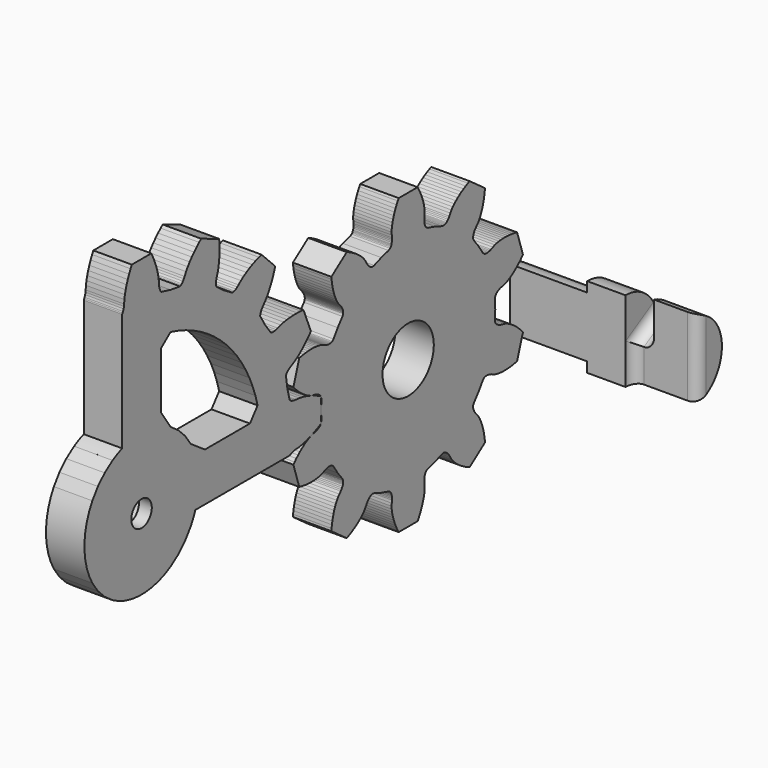
from build123d import *

# Parameters (mm, degrees)
F0_R      = 2.286
F1_DEPTH  = 2.54
F2_R      = 2.286
F2_R_2    = 1.27
F3_DEPTH  = 1.27
F0_R_2    = 3.175
F4_DEPTH  = 3.81
F6_DEPTH  = 7.62
F8_DEPTH  = 10.16
F10_DEPTH = 6.35
F11_W     = 2.032
F11_H     = 3.8688168734
F13_ANGLE = 60
F14_R     = 1.01599


# Not quite as in the source:
# - a fillet or chamfer is up to 0.001 mm smaller than in the source, because OpenCascade refuses the exact size


with BuildPart() as f1:
    # F0 (on Right) → F1 (new body)
    with BuildSketch(Plane.YZ):
        with BuildLine():
            ThreePointArc((-44.3191216143, -0.6106576644), (-44.0103284784, -0.0255231274), (-43.7575535089, 0.5859018))
            ThreePointArc((-43.7575535089, 0.5859018), (-43.4452871465, 1.7648192218), (-43.3401567406, 2.9798518))
            ThreePointArc((-43.3401567406, 2.9798518), (-43.5892848539, 4.8406399116), (-44.3191215541, 6.5703611621))
            Line((-44.3191215541, 6.5703611621), (-44.3195456, 6.5706498))
            Line((-44.3195456, 6.5706498), (-45.0086476, 7.5427078))
            Line((-45.0086476, 7.5427078), (-45.8511656, 8.3852258))
            Line((-45.8511656, 8.3852258), (-46.8232236, 9.0743278))
            Line((-46.8232236, 9.0743278), (-46.8235122379, 9.0747518459))
            ThreePointArc((-46.8235122379, 9.0747518459), (-49.7531295936, 10.0227763208), (-52.8079716, 9.6363198911))
            ThreePointArc((-52.8079716, 9.6363198911), (-53.4193965274, 9.3835449216), (-54.0045310644, 9.0747517857))
            Line((-54.0045310644, 9.0747517857), (-54.0048196, 9.0743278))
            Line((-54.0048196, 9.0743278), (-54.9768776, 8.3852258))
            Line((-54.9768776, 8.3852258), (-55.8196496, 7.5427078))
            Line((-55.8196496, 7.5427078), (-56.5087516, 6.5706498))
            ThreePointArc((-56.5087516, 6.5706498), (-57.4878864594, 2.9798518), (-56.5087516, -0.6109462))
            Line((-56.5087516, -0.6109462), (-55.8196496, -1.5830042))
            Line((-55.8196496, -1.5830042), (-54.9768776, -2.4257762))
            Line((-54.9768776, -2.4257762), (-54.0048196, -3.1148782))
            ThreePointArc((-54.0048196, -3.1148782), (-50.4140216, -4.0940130594), (-46.8232236, -3.1148782))
            Line((-46.8232236, -3.1148782), (-45.8511656, -2.4257762))
            Line((-45.8511656, -2.4257762), (-45.0086476, -1.5830042))
            Line((-45.0086476, -1.5830042), (-44.3195456, -0.6109462))
            Line((-44.3195456, -0.6109462), (-44.3191216143, -0.6106576644))
        make_face()
        with Locations((-50.4140216, 2.9798518)):
            Circle(F0_R, mode=Mode.SUBTRACT)
        with BuildLine():
            Line((-32.0736976, 5.4146958), (-32.3619876, 6.5706498))
            Line((-32.3619876, 6.5706498), (-32.5380096, 7.7489558))
            Line((-32.5380096, 7.7489558), (-32.4712076, 7.8690978))
            Line((-32.4712076, 7.8690978), (-32.3972936, 7.9618078))
            Line((-32.3972936, 7.9618078), (-32.2390516, 8.1065878))
            Line((-32.2390516, 8.1065878), (-32.0721736, 8.2193638))
            Line((-32.0721736, 8.2193638), (-31.8997076, 8.3123278))
            Line((-31.8997076, 8.3123278), (-31.5524896, 8.4901278))
            Line((-31.5524896, 8.4901278), (-31.2159396, 8.7019638))
            Line((-31.2159396, 8.7019638), (-30.8877716, 8.9402158))
            Line((-30.8877716, 8.9402158), (-30.5679856, 9.2015818))
            Line((-30.5679856, 9.2015818), (-30.2560736, 9.4842838))
            Line((-30.2560736, 9.4842838), (-29.9522896, 9.7862898))
            Line((-29.9522896, 9.7862898), (-29.6563796, 10.1068378))
            Line((-29.6563796, 10.1068378), (-29.4399716, 10.3590598))
            Line((-29.4399716, 10.3590598), (-30.3652936, 12.5927358))
            Line((-30.3652936, 12.5927358), (-30.6965096, 12.6181358))
            Line((-30.6965096, 12.6181358), (-31.1323736, 12.6356618))
            Line((-31.1323736, 12.6356618), (-31.5608716, 12.6343918))
            Line((-31.5608716, 12.6343918), (-31.9812416, 12.6135638))
            Line((-31.9812416, 12.6135638), (-32.3922136, 12.5721618))
            Line((-32.3922136, 12.5721618), (-32.7927716, 12.5089158))
            Line((-32.7927716, 12.5089158), (-33.1806296, 12.4205238))
            Line((-33.1806296, 12.4205238), (-33.5517236, 12.3008898))
            Line((-33.5517236, 12.3008898), (-33.7394296, 12.2445018))
            Line((-33.7394296, 12.2445018), (-33.9372956, 12.2064018))
            Line((-33.9372956, 12.2064018), (-34.1514176, 12.1967498))
            Line((-34.1514176, 12.1967498), (-34.2692736, 12.2099578))
            Line((-34.2692736, 12.2099578), (-34.4016076, 12.2478038))
            Line((-34.4016076, 12.2478038), (-35.1102676, 13.2053838))
            Line((-35.1102676, 13.2053838), (-35.7236776, 14.2267178))
            Line((-35.7236776, 14.2267178), (-35.7081836, 14.3633698))
            Line((-35.7081836, 14.3633698), (-35.6754176, 14.4771618))
            Line((-35.6754176, 14.4771618), (-35.5844856, 14.6714718))
            Line((-35.5844856, 14.6714718), (-35.4734876, 14.8398738))
            Line((-35.4734876, 14.8398738), (-35.3495356, 14.9915118))
            Line((-35.3495356, 14.9915118), (-35.0970596, 15.2886918))
            Line((-35.0970596, 15.2886918), (-34.8669356, 15.6130498))
            Line((-34.8669356, 15.6130498), (-34.6550996, 15.9589978))
            Line((-34.6550996, 15.9589978), (-34.4597736, 16.3229798))
            Line((-34.4597736, 16.3229798), (-34.2796876, 16.7032178))
            Line((-34.2796876, 16.7032178), (-34.1145876, 17.0986958))
            Line((-34.1145876, 17.0986958), (-33.9639656, 17.5078898))
            Line((-33.9639656, 17.5078898), (-33.8603336, 17.8236118))
            Line((-33.8603336, 17.8236118), (-35.5702616, 19.5335398))
            Line((-35.5702616, 19.5335398), (-35.8859836, 19.4299078))
            Line((-35.8859836, 19.4299078), (-36.2951776, 19.2792858))
            Line((-36.2951776, 19.2792858), (-36.6906556, 19.1141858))
            Line((-36.6906556, 19.1141858), (-37.0708936, 18.9340998))
            Line((-37.0708936, 18.9340998), (-37.4348756, 18.7387738))
            Line((-37.4348756, 18.7387738), (-37.7808236, 18.5269378))
            Line((-37.7808236, 18.5269378), (-38.1051816, 18.2968138))
            Line((-38.1051816, 18.2968138), (-38.4023616, 18.0443378))
            Line((-38.4023616, 18.0443378), (-38.5539996, 17.9203858))
            Line((-38.5539996, 17.9203858), (-38.7224016, 17.8093878))
            Line((-38.7224016, 17.8093878), (-38.9167116, 17.7184558))
            Line((-38.9167116, 17.7184558), (-39.0305036, 17.6856898))
            Line((-39.0305036, 17.6856898), (-39.1671556, 17.6701958))
            Line((-39.1671556, 17.6701958), (-40.1884896, 18.2836058))
            Line((-40.1884896, 18.2836058), (-41.1460696, 18.9922658))
            Line((-41.1460696, 18.9922658), (-41.1839156, 19.1245998))
            Line((-41.1839156, 19.1245998), (-41.1971236, 19.2424558))
            Line((-41.1971236, 19.2424558), (-41.1874716, 19.4565778))
            Line((-41.1874716, 19.4565778), (-41.1493716, 19.6544438))
            Line((-41.1493716, 19.6544438), (-41.0929836, 19.8421498))
            Line((-41.0929836, 19.8421498), (-40.9733496, 20.2132438))
            Line((-40.9733496, 20.2132438), (-40.8849576, 20.6011018))
            Line((-40.8849576, 20.6011018), (-40.8217116, 21.0016598))
            Line((-40.8217116, 21.0016598), (-40.7803096, 21.4126318))
            Line((-40.7803096, 21.4126318), (-40.7594816, 21.8330018))
            Line((-40.7594816, 21.8330018), (-40.7582116, 22.2614998))
            Line((-40.7582116, 22.2614998), (-40.7757376, 22.6973638))
            Line((-40.7757376, 22.6973638), (-40.8011376, 23.0285798))
            Line((-40.8011376, 23.0285798), (-43.0348136, 23.9539018))
            Line((-43.0348136, 23.9539018), (-43.2870356, 23.7374938))
            Line((-43.2870356, 23.7374938), (-43.6075836, 23.4415838))
            Line((-43.6075836, 23.4415838), (-43.9095896, 23.1377998))
            Line((-43.9095896, 23.1377998), (-44.1922916, 22.8258878))
            Line((-44.1922916, 22.8258878), (-44.4536576, 22.5061018))
            Line((-44.4536576, 22.5061018), (-44.6919096, 22.1779338))
            Line((-44.6919096, 22.1779338), (-44.9037456, 21.8413838))
            Line((-44.9037456, 21.8413838), (-45.0815456, 21.4941658))
            Line((-45.0815456, 21.4941658), (-45.1745096, 21.3216998))
            Line((-45.1745096, 21.3216998), (-45.2872856, 21.1548218))
            Line((-45.2872856, 21.1548218), (-45.4320656, 20.9965798))
            Line((-45.4320656, 20.9965798), (-45.5247756, 20.9226658))
            Line((-45.5247756, 20.9226658), (-45.6449176, 20.8558638))
            Line((-45.6449176, 20.8558638), (-46.8232236, 21.0318858))
            Line((-46.8232236, 21.0318858), (-47.9791776, 21.3201758))
            Line((-47.9791776, 21.3201758), (-48.0647756, 21.4278718))
            Line((-48.0647756, 21.4278718), (-48.1221796, 21.5315038))
            Line((-48.1221796, 21.5315038), (-48.1953316, 21.7331798))
            Line((-48.1953316, 21.7331798), (-48.2357176, 21.9307918))
            Line((-48.2357176, 21.9307918), (-48.2555296, 22.1256098))
            Line((-48.2555296, 22.1256098), (-48.2870256, 22.5142298))
            Line((-48.2870256, 22.5142298), (-48.3538276, 22.9064058))
            Line((-48.3538276, 22.9064058), (-48.4485696, 23.3006138))
            Line((-48.4485696, 23.3006138), (-48.5676956, 23.6963458))
            Line((-48.5676956, 23.6963458), (-48.7091736, 24.0925858))
            Line((-48.7091736, 24.0925858), (-48.8719876, 24.4888258))
            Line((-48.8719876, 24.4888258), (-49.0551216, 24.8848118))
            Line((-49.0551216, 24.8848118), (-49.2052356, 25.1812298))
            Line((-49.2052356, 25.1812298), (-51.6230616, 25.1812298))
            Line((-51.6230616, 25.1812298), (-51.7731756, 24.8848118))
            Line((-51.7731756, 24.8848118), (-51.9560556, 24.4888258))
            Line((-51.9560556, 24.4888258), (-52.1188696, 24.0925858))
            Line((-52.1188696, 24.0925858), (-52.2606016, 23.6963458))
            Line((-52.2606016, 23.6963458), (-52.3797276, 23.3006138))
            Line((-52.3797276, 23.3006138), (-52.4744696, 22.9064058))
            Line((-52.4744696, 22.9064058), (-52.5412716, 22.5142298))
            Line((-52.5412716, 22.5142298), (-52.5727676, 22.1256098))
            Line((-52.5727676, 22.1256098), (-52.5923256, 21.9307918))
            Line((-52.5923256, 21.9307918), (-52.6329656, 21.7331798))
            Line((-52.6329656, 21.7331798), (-52.7058636, 21.5315038))
            Line((-52.7058636, 21.5315038), (-52.7632676, 21.4278718))
            Line((-52.7632676, 21.4278718), (-52.8079716, 21.3303745893))
            Line((-52.8079716, 21.3303745893), (-52.8079716, 16.4029898))
            Line((-52.8079716, 16.4029898), (-52.8079716, 10.8330238))
            Line((-52.8079716, 10.8330238), (-52.8079716, 9.6363198911))
            ThreePointArc((-52.8079716, 9.6363198911), (-49.7531295936, 10.0227763208), (-46.8235122379, 9.0747518459))
            Line((-46.8235122379, 9.0747518459), (-48.0203256, 10.8330238))
            Line((-48.0203256, 10.8330238), (-48.0203256, 16.4029898))
            Line((-48.0203256, 16.4029898), (-46.8232236, 17.3529498))
            Line((-46.8232236, 17.3529498), (-45.8610716, 17.0776138))
            Line((-45.8610716, 17.0776138), (-44.9194936, 16.7380158))
            Line((-44.9194936, 16.7380158), (-44.0030616, 16.3356798))
            Line((-44.0030616, 16.3356798), (-43.1158396, 15.8721298))
            Line((-43.1158396, 15.8721298), (-42.2618916, 15.3499058))
            Line((-42.2618916, 15.3499058), (-41.4452816, 14.7712938))
            Line((-41.4452816, 14.7712938), (-40.6695656, 14.1388338))
            Line((-40.6695656, 14.1388338), (-39.9385536, 13.4553198))
            Line((-39.9385536, 13.4553198), (-39.2550396, 12.7243078))
            Line((-39.2550396, 12.7243078), (-38.6225796, 11.9485918))
            Line((-38.6225796, 11.9485918), (-38.0439676, 11.1319818))
            Line((-38.0439676, 11.1319818), (-37.5217436, 10.2780338))
            Line((-37.5217436, 10.2780338), (-37.0581936, 9.3908118))
            Line((-37.0581936, 9.3908118), (-36.6558576, 8.4743798))
            Line((-36.6558576, 8.4743798), (-36.3162596, 7.5328018))
            Line((-36.3162596, 7.5328018), (-36.0409236, 6.5706498))
            Line((-36.0409236, 6.5706498), (-36.9908836, 5.3735478))
            Line((-36.9908836, 5.3735478), (-42.5608496, 5.3735478))
            Line((-42.5608496, 5.3735478), (-44.3191215541, 6.5703611621))
            ThreePointArc((-44.3191215541, 6.5703611621), (-43.5892848539, 4.8406399116), (-43.3401567406, 2.9798518))
            ThreePointArc((-43.3401567406, 2.9798518), (-43.4452871465, 1.7648192218), (-43.7575535089, 0.5859018))
            Line((-43.7575535089, 0.5859018), (-42.5608496, 0.5859018))
            Line((-42.5608496, 0.5859018), (-36.9908836, 0.5859018))
            Line((-36.9908836, 0.5859018), (-32.0634988107, 0.5859018))
            Line((-32.0634988107, 0.5859018), (-31.9660016, 0.6306058))
            Line((-31.9660016, 0.6306058), (-31.8623696, 0.6880098))
            Line((-31.8623696, 0.6880098), (-31.6606936, 0.7609078))
            Line((-31.6606936, 0.7609078), (-31.4630816, 0.8015478))
            Line((-31.4630816, 0.8015478), (-31.2682636, 0.8211058))
            Line((-31.2682636, 0.8211058), (-30.8796436, 0.8526018))
            Line((-30.8796436, 0.8526018), (-30.4874676, 0.9194038))
            Line((-30.4874676, 0.9194038), (-30.0932596, 1.0141458))
            Line((-30.0932596, 1.0141458), (-29.6975276, 1.1332718))
            Line((-29.6975276, 1.1332718), (-29.3012876, 1.2750038))
            Line((-29.3012876, 1.2750038), (-28.9050476, 1.4378178))
            Line((-28.9050476, 1.4378178), (-28.5090616, 1.6206978))
            Line((-28.5090616, 1.6206978), (-28.2164088746, 1.7689049643))
            Line((-28.2164088746, 1.7689049643), (-28.2126436, 1.775045529))
            Line((-28.2126436, 1.775045529), (-28.2126436, 4.184404071))
            Line((-28.2126436, 4.184404071), (-28.2164088746, 4.1905446357))
            Line((-28.2164088746, 4.1905446357), (-28.5090616, 4.3387518))
            Line((-28.5090616, 4.3387518), (-28.9050476, 4.5218858))
            Line((-28.9050476, 4.5218858), (-29.3012876, 4.6846998))
            Line((-29.3012876, 4.6846998), (-29.6975276, 4.8261778))
            Line((-29.6975276, 4.8261778), (-30.0932596, 4.9453038))
            Line((-30.0932596, 4.9453038), (-30.4874676, 5.0400458))
            Line((-30.4874676, 5.0400458), (-30.8796436, 5.1068478))
            Line((-30.8796436, 5.1068478), (-31.2682636, 5.1383438))
            Line((-31.2682636, 5.1383438), (-31.4630816, 5.1581558))
            Line((-31.4630816, 5.1581558), (-31.6606936, 5.1985418))
            Line((-31.6606936, 5.1985418), (-31.8623696, 5.2716938))
            Line((-31.8623696, 5.2716938), (-31.9660016, 5.3290978))
            Line((-31.9660016, 5.3290978), (-32.0736976, 5.4146958))
        make_face()
    extrude(amount=F1_DEPTH)

    # F2 (on face) → F3 (join)
    with BuildSketch(Plane.YZ.offset(2.54)):
        with BuildLine():
            Line((-54.9768776, -2.4257762), (-54.0048196, -3.1148782))
            ThreePointArc((-54.0048196, -3.1148782), (-50.4140216, -4.0940130594), (-46.8232236, -3.1148782))
            Line((-46.8232236, -3.1148782), (-45.8511656, -2.4257762))
            Line((-45.8511656, -2.4257762), (-45.0086476, -1.5830042))
            Line((-45.0086476, -1.5830042), (-44.3195456, -0.6109462))
            Line((-44.3195456, -0.6109462), (-44.3191216143, -0.6106576644))
            ThreePointArc((-44.3191216143, -0.6106576644), (-44.0103284784, -0.0255231274), (-43.7575535089, 0.5859018))
            Line((-43.7575535089, 0.5859018), (-32.0634988107, 0.5859018))
            Line((-32.0634988107, 0.5859018), (-31.9660016, 0.6306058))
            Line((-31.9660016, 0.6306058), (-31.8623696, 0.6880098))
            Line((-31.8623696, 0.6880098), (-31.6606936, 0.7609078))
            Line((-31.6606936, 0.7609078), (-31.4630816, 0.8015478))
            Line((-31.4630816, 0.8015478), (-31.2682636, 0.8211058))
            Line((-31.2682636, 0.8211058), (-30.8796436, 0.8526018))
            Line((-30.8796436, 0.8526018), (-30.4874676, 0.9194038))
            Line((-30.4874676, 0.9194038), (-30.0932596, 1.0141458))
            Line((-30.0932596, 1.0141458), (-29.6975276, 1.1332718))
            Line((-29.6975276, 1.1332718), (-29.3012876, 1.2750038))
            Line((-29.3012876, 1.2750038), (-28.9050476, 1.4378178))
            Line((-28.9050476, 1.4378178), (-28.5090616, 1.6206978))
            Line((-28.5090616, 1.6206978), (-28.2164088746, 1.7689049643))
            Line((-28.2164088746, 1.7689049643), (-28.2126436, 1.775045529))
            Line((-28.2126436, 1.775045529), (-28.2126436, 4.184404071))
            Line((-28.2126436, 4.184404071), (-28.2164088746, 4.1905446357))
            Line((-28.2164088746, 4.1905446357), (-28.5090616, 4.3387518))
            Line((-28.5090616, 4.3387518), (-28.9050476, 4.5218858))
            Line((-28.9050476, 4.5218858), (-29.3012876, 4.6846998))
            Line((-29.3012876, 4.6846998), (-29.6975276, 4.8261778))
            Line((-29.6975276, 4.8261778), (-30.0932596, 4.9453038))
            Line((-30.0932596, 4.9453038), (-30.4874676, 5.0400458))
            Line((-30.4874676, 5.0400458), (-30.8796436, 5.1068478))
            Line((-30.8796436, 5.1068478), (-31.2682636, 5.1383438))
            Line((-31.2682636, 5.1383438), (-31.4630816, 5.1581558))
            Line((-31.4630816, 5.1581558), (-31.6606936, 5.1985418))
            Line((-31.6606936, 5.1985418), (-31.8623696, 5.2716938))
            Line((-31.8623696, 5.2716938), (-31.9660016, 5.3290978))
            Line((-31.9660016, 5.3290978), (-32.0736976, 5.4146958))
            Line((-32.0736976, 5.4146958), (-32.3619876, 6.5706498))
            Line((-32.3619876, 6.5706498), (-32.5380096, 7.7489558))
            Line((-32.5380096, 7.7489558), (-32.4712076, 7.8690978))
            Line((-32.4712076, 7.8690978), (-32.3972936, 7.9618078))
            Line((-32.3972936, 7.9618078), (-32.2390516, 8.1065878))
            Line((-32.2390516, 8.1065878), (-32.0721736, 8.2193638))
            Line((-32.0721736, 8.2193638), (-31.8997076, 8.3123278))
            Line((-31.8997076, 8.3123278), (-31.5524896, 8.4901278))
            Line((-31.5524896, 8.4901278), (-31.2159396, 8.7019638))
            Line((-31.2159396, 8.7019638), (-30.8877716, 8.9402158))
            Line((-30.8877716, 8.9402158), (-30.5679856, 9.2015818))
            Line((-30.5679856, 9.2015818), (-30.2560736, 9.4842838))
            Line((-30.2560736, 9.4842838), (-29.9522896, 9.7862898))
            Line((-29.9522896, 9.7862898), (-29.6563796, 10.1068378))
            Line((-29.6563796, 10.1068378), (-29.4399716, 10.3590598))
            Line((-29.4399716, 10.3590598), (-30.3652936, 12.5927358))
            Line((-30.3652936, 12.5927358), (-30.6965096, 12.6181358))
            Line((-30.6965096, 12.6181358), (-31.1323736, 12.6356618))
            Line((-31.1323736, 12.6356618), (-31.5608716, 12.6343918))
            Line((-31.5608716, 12.6343918), (-31.9812416, 12.6135638))
            Line((-31.9812416, 12.6135638), (-32.3922136, 12.5721618))
            Line((-32.3922136, 12.5721618), (-32.7927716, 12.5089158))
            Line((-32.7927716, 12.5089158), (-33.1806296, 12.4205238))
            Line((-33.1806296, 12.4205238), (-33.5517236, 12.3008898))
            Line((-33.5517236, 12.3008898), (-33.7394296, 12.2445018))
            Line((-33.7394296, 12.2445018), (-33.9372956, 12.2064018))
            Line((-33.9372956, 12.2064018), (-34.1514176, 12.1967498))
            Line((-34.1514176, 12.1967498), (-34.2692736, 12.2099578))
            Line((-34.2692736, 12.2099578), (-34.4016076, 12.2478038))
            Line((-34.4016076, 12.2478038), (-35.1102676, 13.2053838))
            Line((-35.1102676, 13.2053838), (-35.7236776, 14.2267178))
            Line((-35.7236776, 14.2267178), (-35.7081836, 14.3633698))
            Line((-35.7081836, 14.3633698), (-35.6754176, 14.4771618))
            Line((-35.6754176, 14.4771618), (-35.5844856, 14.6714718))
            Line((-35.5844856, 14.6714718), (-35.4734876, 14.8398738))
            Line((-35.4734876, 14.8398738), (-35.3495356, 14.9915118))
            Line((-35.3495356, 14.9915118), (-35.0970596, 15.2886918))
            Line((-35.0970596, 15.2886918), (-34.8669356, 15.6130498))
            Line((-34.8669356, 15.6130498), (-34.6550996, 15.9589978))
            Line((-34.6550996, 15.9589978), (-34.4597736, 16.3229798))
            Line((-34.4597736, 16.3229798), (-34.2796876, 16.7032178))
            Line((-34.2796876, 16.7032178), (-34.1145876, 17.0986958))
            Line((-34.1145876, 17.0986958), (-33.9639656, 17.5078898))
            Line((-33.9639656, 17.5078898), (-33.8603336, 17.8236118))
            Line((-33.8603336, 17.8236118), (-35.5702616, 19.5335398))
            Line((-35.5702616, 19.5335398), (-35.8859836, 19.4299078))
            Line((-35.8859836, 19.4299078), (-36.2951776, 19.2792858))
            Line((-36.2951776, 19.2792858), (-36.6906556, 19.1141858))
            Line((-36.6906556, 19.1141858), (-37.0708936, 18.9340998))
            Line((-37.0708936, 18.9340998), (-37.4348756, 18.7387738))
            Line((-37.4348756, 18.7387738), (-37.7808236, 18.5269378))
            Line((-37.7808236, 18.5269378), (-38.1051816, 18.2968138))
            Line((-38.1051816, 18.2968138), (-38.4023616, 18.0443378))
            Line((-38.4023616, 18.0443378), (-38.5539996, 17.9203858))
            Line((-38.5539996, 17.9203858), (-38.7224016, 17.8093878))
            Line((-38.7224016, 17.8093878), (-38.9167116, 17.7184558))
            Line((-38.9167116, 17.7184558), (-39.0305036, 17.6856898))
            Line((-39.0305036, 17.6856898), (-39.1671556, 17.6701958))
            Line((-39.1671556, 17.6701958), (-40.1884896, 18.2836058))
            Line((-40.1884896, 18.2836058), (-41.1460696, 18.9922658))
            Line((-41.1460696, 18.9922658), (-41.1839156, 19.1245998))
            Line((-41.1839156, 19.1245998), (-41.1971236, 19.2424558))
            Line((-41.1971236, 19.2424558), (-41.1874716, 19.4565778))
            Line((-41.1874716, 19.4565778), (-41.1493716, 19.6544438))
            Line((-41.1493716, 19.6544438), (-41.0929836, 19.8421498))
            Line((-41.0929836, 19.8421498), (-40.9733496, 20.2132438))
            Line((-40.9733496, 20.2132438), (-40.8849576, 20.6011018))
            Line((-40.8849576, 20.6011018), (-40.8217116, 21.0016598))
            Line((-40.8217116, 21.0016598), (-40.7803096, 21.4126318))
            Line((-40.7803096, 21.4126318), (-40.7594816, 21.8330018))
            Line((-40.7594816, 21.8330018), (-40.7582116, 22.2614998))
            Line((-40.7582116, 22.2614998), (-40.7757376, 22.6973638))
            Line((-40.7757376, 22.6973638), (-40.8011376, 23.0285798))
            Line((-40.8011376, 23.0285798), (-43.0348136, 23.9539018))
            Line((-43.0348136, 23.9539018), (-43.2870356, 23.7374938))
            Line((-43.2870356, 23.7374938), (-43.6075836, 23.4415838))
            Line((-43.6075836, 23.4415838), (-43.9095896, 23.1377998))
            Line((-43.9095896, 23.1377998), (-44.1922916, 22.8258878))
            Line((-44.1922916, 22.8258878), (-44.4536576, 22.5061018))
            Line((-44.4536576, 22.5061018), (-44.6919096, 22.1779338))
            Line((-44.6919096, 22.1779338), (-44.9037456, 21.8413838))
            Line((-44.9037456, 21.8413838), (-45.0815456, 21.4941658))
            Line((-45.0815456, 21.4941658), (-45.1745096, 21.3216998))
            Line((-45.1745096, 21.3216998), (-45.2872856, 21.1548218))
            Line((-45.2872856, 21.1548218), (-45.4320656, 20.9965798))
            Line((-45.4320656, 20.9965798), (-45.5247756, 20.9226658))
            Line((-45.5247756, 20.9226658), (-45.6449176, 20.8558638))
            Line((-45.6449176, 20.8558638), (-46.8232236, 21.0318858))
            Line((-46.8232236, 21.0318858), (-47.9791776, 21.3201758))
            Line((-47.9791776, 21.3201758), (-48.0647756, 21.4278718))
            Line((-48.0647756, 21.4278718), (-48.1221796, 21.5315038))
            Line((-48.1221796, 21.5315038), (-48.1953316, 21.7331798))
            Line((-48.1953316, 21.7331798), (-48.2357176, 21.9307918))
            Line((-48.2357176, 21.9307918), (-48.2555296, 22.1256098))
            Line((-48.2555296, 22.1256098), (-48.2870256, 22.5142298))
            Line((-48.2870256, 22.5142298), (-48.3538276, 22.9064058))
            Line((-48.3538276, 22.9064058), (-48.4485696, 23.3006138))
            Line((-48.4485696, 23.3006138), (-48.5676956, 23.6963458))
            Line((-48.5676956, 23.6963458), (-48.7091736, 24.0925858))
            Line((-48.7091736, 24.0925858), (-48.8719876, 24.4888258))
            Line((-48.8719876, 24.4888258), (-49.0551216, 24.8848118))
            Line((-49.0551216, 24.8848118), (-49.2052356, 25.1812298))
            Line((-49.2052356, 25.1812298), (-51.6230616, 25.1812298))
            Line((-51.6230616, 25.1812298), (-51.7731756, 24.8848118))
            Line((-51.7731756, 24.8848118), (-51.9560556, 24.4888258))
            Line((-51.9560556, 24.4888258), (-52.1188696, 24.0925858))
            Line((-52.1188696, 24.0925858), (-52.2606016, 23.6963458))
            Line((-52.2606016, 23.6963458), (-52.3797276, 23.3006138))
            Line((-52.3797276, 23.3006138), (-52.4744696, 22.9064058))
            Line((-52.4744696, 22.9064058), (-52.5412716, 22.5142298))
            Line((-52.5412716, 22.5142298), (-52.5727676, 22.1256098))
            Line((-52.5727676, 22.1256098), (-52.5923256, 21.9307918))
            Line((-52.5923256, 21.9307918), (-52.6329656, 21.7331798))
            Line((-52.6329656, 21.7331798), (-52.7058636, 21.5315038))
            Line((-52.7058636, 21.5315038), (-52.7632676, 21.4278718))
            Line((-52.7632676, 21.4278718), (-52.8079716, 21.3303745893))
            Line((-52.8079716, 21.3303745893), (-52.8079716, 9.6363198911))
            ThreePointArc((-52.8079716, 9.6363198911), (-53.4193965274, 9.3835449216), (-54.0045310644, 9.0747517857))
            Line((-54.0045310644, 9.0747517857), (-54.0048196, 9.0743278))
            Line((-54.0048196, 9.0743278), (-54.9768776, 8.3852258))
            Line((-54.9768776, 8.3852258), (-55.8196496, 7.5427078))
            Line((-55.8196496, 7.5427078), (-56.5087516, 6.5706498))
            ThreePointArc((-56.5087516, 6.5706498), (-57.4878864594, 2.9798518), (-56.5087516, -0.6109462))
            Line((-56.5087516, -0.6109462), (-55.8196496, -1.5830042))
            Line((-55.8196496, -1.5830042), (-54.9768776, -2.4257762))
        make_face()
        with Locations((-50.4140216, 2.9798518)):
            Circle(F2_R, mode=Mode.SUBTRACT)
        Polygon((-42.5608496, 5.3735478), (-44.3195456, 6.5706498), (-45.0086476, 7.5427078), (-45.8511656, 8.3852258), (-46.8232236, 9.0743278), (-46.8235122379, 9.0747518459), (-48.0203256, 10.8330238), (-48.0203256, 16.4029898), (-46.8232236, 17.3529498), (-45.8610716, 17.0776138), (-44.9194936, 16.7380158), (-44.0030616, 16.3356798), (-43.1158396, 15.8721298), (-42.2618916, 15.3499058), (-41.4452816, 14.7712938), (-40.6695656, 14.1388338), (-39.9385536, 13.4553198), (-39.2550396, 12.7243078), (-38.6225796, 11.9485918), (-38.0439676, 11.1319818), (-37.5217436, 10.2780338), (-37.0581936, 9.3908118), (-36.6558576, 8.4743798), (-36.3162596, 7.5328018), (-36.0409236, 6.5706498), (-36.9908836, 5.3735478), align=None, mode=Mode.SUBTRACT)
        with Locations((-50.4140216, 2.9798518)):
            Circle(F2_R)
        with Locations((-50.4140216, 2.9798518)):
            Circle(F2_R_2, mode=Mode.SUBTRACT)
    extrude(amount=F3_DEPTH)


with BuildPart() as f4:
    # F0 (on Right) → F4 (new body)
    with BuildSketch(Plane.YZ):
        Polygon((-28.2362656, 4.2229278), (-28.2164088746, 4.1905446357), (-28.2126436, 4.1886378), (-28.2126436, 4.184404071), (-28.1819096, 4.1342818), (-28.1389836, 3.9173658), (-28.1798776, 2.9798518), (-28.1389836, 2.0420838), (-28.1819096, 1.8251678), (-28.2126436, 1.775045529), (-28.2126436, 1.7708118), (-28.2164088746, 1.7689049643), (-28.2362656, 1.7365218), (-28.2929076, 1.6704818), (-28.3505656, 1.6166338), (-28.4089856, 1.5706598), (-28.5278576, 1.4957298), (-28.6487616, 1.4365478), (-28.7709356, 1.3893038), (-28.8946336, 1.3512038), (-29.1448236, 1.2981178), (-29.3942516, 1.2386818), (-29.6380916, 1.1431778), (-29.8781216, 1.0253218), (-30.1148496, 0.8894318), (-30.3480216, 0.7372858), (-30.5776376, 0.5704078), (-30.8034436, 0.3893058), (-31.0249316, 0.1947418), (-31.2421016, -0.0125222), (-31.4546996, -0.2319782), (-31.6111636, -0.4046982), (-30.8852316, -2.6386282), (-30.6573936, -2.6863802), (-30.3561496, -2.7392122), (-30.0587156, -2.7790902), (-29.7650916, -2.8062682), (-29.4760396, -2.8199842), (-29.1920676, -2.8202382), (-28.9141916, -2.8062682), (-28.6426656, -2.7770582), (-28.3792676, -2.7310842), (-28.1257756, -2.6650442), (-27.8890476, -2.5664922), (-27.6553676, -2.4626062), (-27.5331936, -2.4206962), (-27.4064476, -2.3871682), (-27.2738596, -2.3638002), (-27.1336516, -2.3546562), (-27.0592296, -2.3574502), (-26.9809976, -2.3671022), (-26.8964156, -2.3874222), (-26.8004036, -2.4270462), (-26.6380976, -2.5774142), (-26.1199376, -3.3599882), (-25.5357376, -4.0945562), (-25.4430276, -4.2952162), (-25.4348996, -4.3988482), (-25.4417576, -4.4854622), (-25.4567436, -4.5631862), (-25.4770636, -4.6345602), (-25.5291336, -4.7653702), (-25.5921256, -4.8839882), (-25.6632456, -4.9942242), (-25.7409696, -5.0976022), (-25.9121656, -5.2875942), (-26.0790436, -5.4821582), (-26.2200136, -5.7028842), (-26.3452356, -5.9393582), (-26.4567416, -6.1885322), (-26.5560556, -6.4486282), (-26.6436856, -6.7186302), (-26.7196316, -6.9977762), (-26.7846556, -7.2853042), (-26.8387576, -7.5807062), (-26.8816836, -7.8834742), (-26.9065756, -8.1148682), (-25.0061476, -9.4956122), (-24.7938036, -9.4003622), (-24.5192296, -9.2659962), (-24.2548156, -9.1232482), (-24.0015776, -8.9726262), (-23.7595156, -8.8138762), (-23.5296456, -8.6472522), (-23.3129836, -8.4725002), (-23.1105456, -8.2893662), (-22.9243636, -8.0973422), (-22.7582476, -7.8949042), (-22.6246436, -7.6762102), (-22.4968816, -7.4547222), (-22.4224596, -7.3488042), (-22.3396556, -7.2472042), (-22.2461836, -7.1504302), (-22.1379796, -7.0605142), (-22.0762576, -7.0191122), (-22.0071696, -6.9810122), (-21.9269056, -6.9477382), (-21.8258136, -6.9233542), (-21.6061036, -6.9495162), (-20.7270096, -7.2779382), (-19.8227696, -7.5288902), (-19.6297296, -7.6368402), (-19.5621656, -7.7160882), (-19.5169536, -7.7902562), (-19.4834256, -7.8616302), (-19.4577716, -7.9314802), (-19.4232276, -8.0678782), (-19.4041776, -8.2009742), (-19.3970656, -8.3317842), (-19.3990976, -8.4610702), (-19.4257676, -8.7155782), (-19.4465956, -8.9711022), (-19.4308476, -9.2324682), (-19.3932556, -9.4973902), (-19.3371216, -9.7643442), (-19.2644776, -10.0330762), (-19.1765936, -10.3030782), (-19.0739776, -10.5735882), (-18.9576456, -10.8446062), (-18.8275976, -11.1151162), (-18.6843416, -11.3853722), (-18.5685176, -11.5873022), (-16.2197796, -11.5873022), (-16.1037016, -11.3853722), (-15.9606996, -11.1151162), (-15.8306516, -10.8446062), (-15.7140656, -10.5735882), (-15.6117036, -10.3030782), (-15.5238196, -10.0330762), (-15.4511756, -9.7643442), (-15.3950416, -9.4973902), (-15.3571956, -9.2324682), (-15.3417016, -8.9711022), (-15.3622756, -8.7155782), (-15.3889456, -8.4610702), (-15.3912316, -8.3317842), (-15.3838656, -8.2009742), (-15.3650696, -8.0678782), (-15.3305256, -7.9314802), (-15.3048716, -7.8616302), (-15.2713436, -7.7902562), (-15.2258776, -7.7160882), (-15.1585676, -7.6368402), (-14.9655276, -7.5288902), (-14.0610336, -7.2779382), (-13.1819396, -6.9495162), (-12.9624836, -6.9233542), (-12.8613916, -6.9477382), (-12.7811276, -6.9810122), (-12.7117856, -7.0191122), (-12.6500636, -7.0605142), (-12.5421136, -7.1504302), (-12.4486416, -7.2472042), (-12.3658376, -7.3488042), (-12.2914156, -7.4547222), (-12.1633996, -7.6762102), (-12.0300496, -7.8949042), (-11.8636796, -8.0973422), (-11.6774976, -8.2893662), (-11.4750596, -8.4725002), (-11.2583976, -8.6472522), (-11.0287816, -8.8138762), (-10.7867196, -8.9726262), (-10.5332276, -9.1232482), (-10.2690676, -9.2659962), (-9.9944936, -9.4003622), (-9.7818956, -9.4956122), (-7.8817216, -8.1148682), (-7.9066136, -7.8834742), (-7.9495396, -7.5807062), (-8.0033876, -7.2853042), (-8.0684116, -6.9977762), (-8.1446116, -6.7186302), (-8.2322416, -6.4486282), (-8.3313016, -6.1885322), (-8.4430616, -5.9393582), (-8.5680296, -5.7028842), (-8.7092536, -5.4821582), (-8.8761316, -5.2875942), (-9.0473276, -5.0976022), (-9.1247976, -4.9942242), (-9.1959176, -4.8839882), (-9.2589096, -4.7653702), (-9.3109796, -4.6345602), (-9.3315536, -4.5631862), (-9.3462856, -4.4854622), (-9.3531436, -4.3988482), (-9.3452696, -4.2952162), (-9.2525596, -4.0945562), (-8.6683596, -3.3599882), (-8.1501996, -2.5774142), (-7.9878936, -2.4270462), (-7.8918816, -2.3874222), (-7.8072996, -2.3671022), (-7.7288136, -2.3574502), (-7.6546456, -2.3546562), (-7.5141836, -2.3638002), (-7.3818496, -2.3871682), (-7.2551036, -2.4206962), (-7.1326756, -2.4626062), (-6.8989956, -2.5664922), (-6.6625216, -2.6650442), (-6.4090296, -2.7310842), (-6.1453776, -2.7770582), (-5.8741056, -2.8062682), (-5.5959756, -2.8202382), (-5.3122576, -2.8199842), (-5.0232056, -2.8062682), (-4.7295816, -2.7790902), (-4.4318936, -2.7392122), (-4.1309036, -2.6863802), (-3.9028116, -2.6386282), (-3.1771336, -0.4046982), (-3.3333436, -0.2319782), (-3.5459416, -0.0125222), (-3.7633656, 0.1947418), (-3.9848536, 0.3893058), (-4.2106596, 0.5704078), (-4.4400216, 0.7372858), (-4.6731936, 0.8894318), (-4.9099216, 1.0253218), (-5.1502056, 1.1431778), (-5.3940456, 1.2386818), (-5.6434736, 1.2981178), (-5.8936636, 1.3512038), (-6.0171076, 1.3893038), (-6.1395356, 1.4365478), (-6.2601856, 1.4957298), (-6.3790576, 1.5706598), (-6.4377316, 1.6166338), (-6.4953896, 1.6704818), (-6.5517776, 1.7365218), (-6.6061336, 1.8251678), (-6.6493136, 2.0420838), (-6.6084196, 2.9798518), (-6.6493136, 3.9173658), (-6.6061336, 4.1342818), (-6.5517776, 4.2229278), (-6.4953896, 4.2889678), (-6.4377316, 4.3430698), (-6.3790576, 4.3887898), (-6.2601856, 4.4639738), (-6.1395356, 4.5229018), (-6.0171076, 4.5703998), (-5.8936636, 4.6082458), (-5.6434736, 4.6615858), (-5.3940456, 4.7207678), (-5.1502056, 4.8165258), (-4.9099216, 4.9341278), (-4.6731936, 5.0700178), (-4.4400216, 5.2221638), (-4.2106596, 5.3892958), (-3.9848536, 5.5703978), (-3.7633656, 5.7647078), (-3.5459416, 5.9719718), (-3.3333436, 6.1916818), (-3.1771336, 6.3644018), (-3.9028116, 8.5980778), (-4.1309036, 8.6460838), (-4.4318936, 8.6986618), (-4.7295816, 8.7387938), (-5.0232056, 8.7657178), (-5.3122576, 8.7796878), (-5.5959756, 8.7799418), (-5.8741056, 8.7657178), (-6.1453776, 8.7367618), (-6.4090296, 8.6907878), (-6.6625216, 8.6247478), (-6.8989956, 8.5261958), (-7.1326756, 8.4220558), (-7.2551036, 8.3801458), (-7.3818496, 8.3466178), (-7.5141836, 8.3235038), (-7.6546456, 8.3141058), (-7.7288136, 8.3168998), (-7.8072996, 8.3268058), (-7.8918816, 8.3468718), (-7.9878936, 8.3867498), (-8.1501996, 8.5368638), (-8.6683596, 9.3194378), (-9.2525596, 10.0540058), (-9.3452696, 10.2546658), (-9.3531436, 10.3582978), (-9.3462856, 10.4451658), (-9.3315536, 10.5226358), (-9.3109796, 10.5942638), (-9.2589096, 10.7248198), (-9.1959176, 10.8436918), (-9.1247976, 10.9536738), (-9.0473276, 11.0570518), (-8.8761316, 11.2472978), (-8.7092536, 11.4418618), (-8.5680296, 11.6625878), (-8.4430616, 11.8988078), (-8.3313016, 12.1479818), (-8.2322416, 12.4080778), (-8.1446116, 12.6780798), (-8.0684116, 12.9572258), (-8.0033876, 13.2447538), (-7.9495396, 13.5401558), (-7.9066136, 13.8429238), (-7.8817216, 14.0743178), (-9.7818956, 15.4550618), (-9.9944936, 15.3598118), (-10.2690676, 15.2254458), (-10.5332276, 15.0829518), (-10.7867196, 14.9320758), (-11.0287816, 14.7735798), (-11.2583976, 14.6069558), (-11.4750596, 14.4322038), (-11.6774976, 14.2490698), (-11.8636796, 14.0567918), (-12.0300496, 13.8546078), (-12.1633996, 13.6356598), (-12.2914156, 13.4141718), (-12.3658376, 13.3085078), (-12.4486416, 13.2066538), (-12.5421136, 13.1101338), (-12.6500636, 13.0202178), (-12.7117856, 12.9788158), (-12.7811276, 12.9404618), (-12.8613916, 12.9071878), (-12.9624836, 12.8828038), (-13.1819396, 12.9089658), (-14.0610336, 13.2376418), (-14.9655276, 13.4885938), (-15.1585676, 13.5965438), (-15.2258776, 13.6755378), (-15.2713436, 13.7497058), (-15.3048716, 13.8213338), (-15.3305256, 13.8911838), (-15.3650696, 14.0273278), (-15.3838656, 14.1604238), (-15.3912316, 14.2914878), (-15.3889456, 14.4205198), (-15.3622756, 14.6750278), (-15.3417016, 14.9305518), (-15.3571956, 15.1919178), (-15.3950416, 15.4568398), (-15.4511756, 15.7240478), (-15.5238196, 15.9927798), (-15.6117036, 16.2625278), (-15.7140656, 16.5332918), (-15.8306516, 16.8040558), (-15.9606996, 17.0748198), (-16.1037016, 17.3448218), (-16.2197796, 17.5467518), (-18.5685176, 17.5467518), (-18.6843416, 17.3448218), (-18.8275976, 17.0748198), (-18.9576456, 16.8040558), (-19.0739776, 16.5332918), (-19.1765936, 16.2625278), (-19.2644776, 15.9927798), (-19.3371216, 15.7240478), (-19.3932556, 15.4568398), (-19.4308476, 15.1919178), (-19.4465956, 14.9305518), (-19.4257676, 14.6750278), (-19.3990976, 14.4205198), (-19.3970656, 14.2914878), (-19.4041776, 14.1604238), (-19.4232276, 14.0273278), (-19.4577716, 13.8911838), (-19.4834256, 13.8213338), (-19.5169536, 13.7497058), (-19.5621656, 13.6755378), (-19.6297296, 13.5965438), (-19.8227696, 13.4885938), (-20.7270096, 13.2376418), (-21.6061036, 12.9089658), (-21.8258136, 12.8828038), (-21.9269056, 12.9071878), (-22.0071696, 12.9404618), (-22.0762576, 12.9788158), (-22.1379796, 13.0202178), (-22.2461836, 13.1101338), (-22.3396556, 13.2066538), (-22.4224596, 13.3085078), (-22.4968816, 13.4141718), (-22.6246436, 13.6356598), (-22.7582476, 13.8546078), (-22.9243636, 14.0567918), (-23.1105456, 14.2490698), (-23.3129836, 14.4322038), (-23.5296456, 14.6069558), (-23.7595156, 14.7735798), (-24.0015776, 14.9320758), (-24.2548156, 15.0829518), (-24.5192296, 15.2254458), (-24.7938036, 15.3598118), (-25.0061476, 15.4550618), (-26.9065756, 14.0743178), (-26.8816836, 13.8429238), (-26.8387576, 13.5401558), (-26.7846556, 13.2447538), (-26.7196316, 12.9572258), (-26.6436856, 12.6780798), (-26.5560556, 12.4080778), (-26.4567416, 12.1479818), (-26.3452356, 11.8988078), (-26.2200136, 11.6625878), (-26.0790436, 11.4418618), (-25.9121656, 11.2472978), (-25.7409696, 11.0570518), (-25.6632456, 10.9536738), (-25.5921256, 10.8436918), (-25.5291336, 10.7248198), (-25.4770636, 10.5942638), (-25.4567436, 10.5226358), (-25.4417576, 10.4451658), (-25.4348996, 10.3582978), (-25.4430276, 10.2546658), (-25.5357376, 10.0540058), (-26.1199376, 9.3194378), (-26.6380976, 8.5368638), (-26.8004036, 8.3867498), (-26.8964156, 8.3468718), (-26.9809976, 8.3268058), (-27.0592296, 8.3168998), (-27.1336516, 8.3141058), (-27.2738596, 8.3235038), (-27.4064476, 8.3466178), (-27.5331936, 8.3801458), (-27.6553676, 8.4220558), (-27.8890476, 8.5261958), (-28.1257756, 8.6247478), (-28.3792676, 8.6907878), (-28.6426656, 8.7367618), (-28.9141916, 8.7657178), (-29.1920676, 8.7799418), (-29.4760396, 8.7796878), (-29.7650916, 8.7657178), (-30.0587156, 8.7387938), (-30.3561496, 8.6986618), (-30.6573936, 8.6460838), (-30.8852316, 8.5980778), (-31.6111636, 6.3644018), (-31.4546996, 6.1916818), (-31.2421016, 5.9719718), (-31.0249316, 5.7647078), (-30.8034436, 5.5703978), (-30.5776376, 5.3892958), (-30.3480216, 5.2221638), (-30.1148496, 5.0700178), (-29.8781216, 4.9341278), (-29.6380916, 4.8165258), (-29.3942516, 4.7207678), (-29.1448236, 4.6615858), (-28.8946336, 4.6082458), (-28.7709356, 4.5703998), (-28.6487616, 4.5229018), (-28.5278576, 4.4639738), (-28.4089856, 4.3887898), (-28.3505656, 4.3430698), (-28.2929076, 4.2889678), align=None)
        with Locations((-17.3940216, 2.9798518)):
            Circle(F0_R_2, mode=Mode.SUBTRACT)
    extrude(amount=F4_DEPTH)


with BuildPart() as f6:
    # F5 (on Right) → F6 (new body)
    with BuildSketch(Plane.YZ):
        with BuildLine():
            ThreePointArc((0, -3), (2.1213203436, -2.1213203436), (3, 0))
            ThreePointArc((3, 0), (2.1213203436, 2.1213203436), (0, 3))
            Line((0, 3), (0, -3))
        make_face()
    extrude(amount=F6_DEPTH)

    # F7 (on face) → F8 (join)
    with BuildSketch(Plane.YZ.offset(7.62)):
        with BuildLine():
            ThreePointArc((0, 3), (3, 0), (0, -3))
            Line((0, -3), (0, -4))
            ThreePointArc((0, -4), (2.8284271247, -2.8284271247), (4, 0))
            ThreePointArc((4, 0), (2.8284271247, 2.8284271247), (0, 4))
            Line((0, 4), (0, 3))
        make_face()
        with BuildLine():
            Line((0, 3), (0, -3))
            ThreePointArc((0, -3), (3, 0), (0, 3))
        make_face()
    extrude(amount=F8_DEPTH)

    # F9 (on face) → F10 (cut)
    with BuildSketch(Plane.YZ.offset(17.78)):
        with BuildLine():
            ThreePointArc((1.016, 3.8688168734), (0.5122169981, 3.9670686592), (0, 4))
            Line((0, 4), (0, -4))
            ThreePointArc((0, -4), (0.5122169981, -3.9670686592), (1.016, -3.8688168734))
            Line((1.016, -3.8688168734), (1.016, 3.8688168734))
        make_face()
    extrude(amount=-F10_DEPTH, mode=Mode.SUBTRACT)

    # F11 (on face) → F13 (revolve, cut)
    with BuildSketch(Plane.XZ.offset(-1.016)):
        with Locations((12.446, 1.9344084367)):
            Rectangle(F11_W, F11_H)
    revolve(axis=Axis((5.715, 0, 0), (-1, 0, 0)), revolution_arc=F13_ANGLE, mode=Mode.SUBTRACT)

    # F14 (radius 1.016 in the source; OpenCascade refuses exactly that, so slightly less here)
    f14_edges = [f6.edges().sort_by_distance(p)[0] for p in [
        (11.43, 2.437247, 0.233969),
        (13.462, 2.437247, 0.233969),
        (11.43, 1.016, -2.227702),
        (17.78, 1.016, 0),
    ]]
    fillet(f14_edges, radius=F14_R)


solid = Compound([f1.part, f4.part, f6.part])
